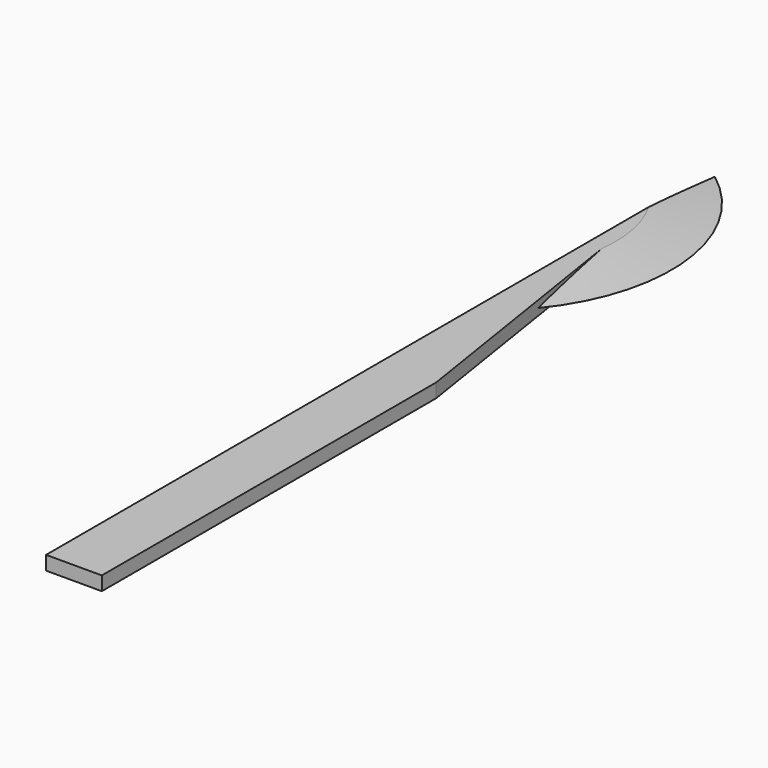
from build123d import *

# Parameters (mm, degrees)
F1_DEPTH   = 1.27
F2_SIZE2   = 0.635
F2_SIZE    = 5.08
F2_2_SIZE2 = 0.63499
F2_2_SIZE  = 5.07999


# Not quite as in the source:
# - a fillet or chamfer is up to 0.001 mm smaller than in the source, because OpenCascade refuses the exact size


with BuildPart() as f1:
    # F0 (on Top) → F1 (new body)
    with BuildSketch(Plane.XY):
        with BuildLine():
            Line((-36.8330654015, 25.4), (-36.8330654015, 0))
            Line((-36.8330654015, 0), (-31.7530654015, 0))
            Line((-31.7530654015, 0), (-31.7530654015, 25.4))
            Line((-31.7530654015, 25.4), (-31.7530654015, 38.1))
            Line((-31.7530654015, 38.1), (-34.0151443949, 52.5287568289))
            ThreePointArc((-34.0151443949, 52.5287568289), (-30.3739911163, 64.9655644869), (-36.8330654015, 76.2))
            Line((-36.8330654015, 76.2), (-36.8330654015, 25.4))
        make_face()
    extrude(amount=F1_DEPTH)

    # F2
    f2_edges = [f1.edges().sort_by_distance(p)[0] for p in [
        (-30.373991, 64.965564, 1.27),
    ]]
    f2_side = f1.faces().sort_by_distance((-34.308504, 37.141649, 1.27))[0]
    chamfer(f2_edges, length=F2_SIZE, length2=F2_SIZE2, reference=f2_side)

    # F2#2 (size 5.08 and 0.635 in the source; OpenCascade refuses exactly that, so slightly less here)
    f2_2_edges = [f1.edges().sort_by_distance(p)[0] for p in [
        (-30.373991, 64.965564, 0),
    ]]
    f2_2_side = f1.faces().sort_by_distance((-34.308504, 37.141649, 0))[0]
    chamfer(f2_2_edges, length=F2_2_SIZE, length2=F2_2_SIZE2, reference=f2_2_side)


solid = f1.part
